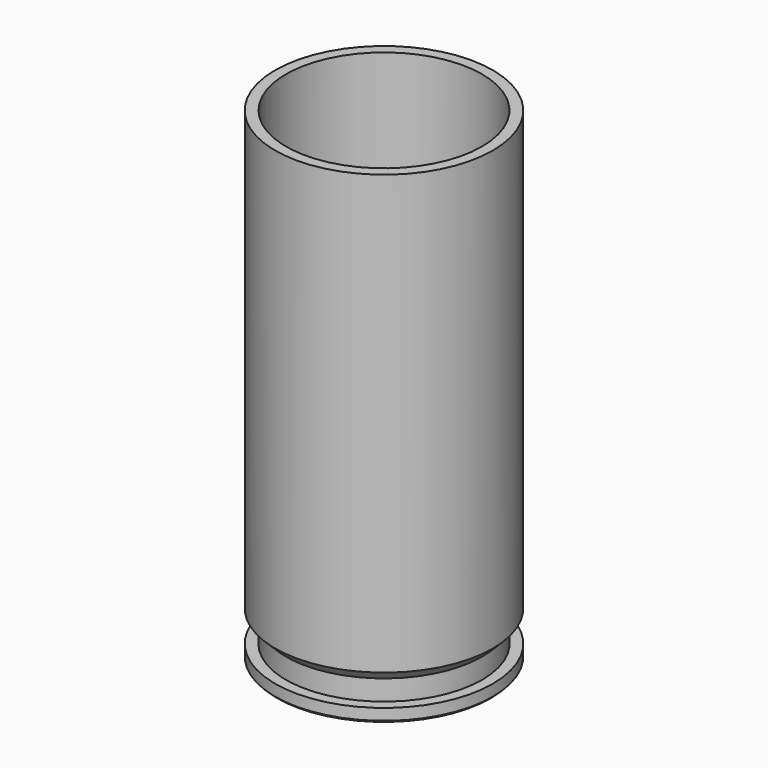
from build123d import *

# Parameters (mm, degrees)
F2_T        = -1.27
F3_SIZE     = 0.254
F4_R        = 6.9696549561
F4_R_2      = 6.3199888533
F5_DEPTH    = 0.254
F7_S5_R     = 11.5270866081
F7_T6_DEPTH = 20


# Not quite as in the source:
# - a fillet or chamfer that OpenCascade refuses, or shapes differently, is made with other operations: its cross-section is extruded or revolved along the edge and cut away or added


with BuildPart() as f1:
    # F0 (on Front) → F1 (revolve)
    with BuildSketch(Plane.XZ):
        Polygon((0, 56.7248165607), (0, 0), (12.7805937082, 0), (12.7805937082, 1.5856500249), (11.5270866081, 1.5856500249), (11.5270866081, 2.6958733797), (12.7805937082, 2.6958733797), (12.7805937082, 56.7248165607), align=None)
    revolve(axis=Axis((0, 0, 24.1605676711), (0, 0, -1)))

    # F2
    f2_openings = [f1.faces().sort_by_distance(p)[0] for p in [
        (0, 0, 56.724817),
    ]]
    offset(amount=F2_T, openings=f2_openings, kind=Kind.INTERSECTION)

    # F3
    f3_edges = [f1.edges().sort_by_distance(p)[0] for p in [
        (-12.780594, 0, 0),
    ]]
    chamfer(f3_edges, length=F3_SIZE)

    # F4 (on face) → F5 (cut)
    with BuildSketch(Plane(origin=(0, 0, 0), x_dir=(1, 0, 0), z_dir=(0, 0, -1))):
        Circle(F4_R)
        Circle(F4_R_2, mode=Mode.SUBTRACT)
    extrude(amount=-F5_DEPTH, mode=Mode.SUBTRACT)

    # F6: fillet of radius 0.762 on 2 edges, made by hand

    # F6_s1 → F6_t2 (revolve, cut)
    with BuildSketch(Plane.XZ):
        with BuildLine():
            ThreePointArc((6.3199888533, 0.254), (6.0631127843, 0.066392352), (5.752027587, 0))
            Line((5.752027587, 0), (6.3199888533, 0))
            Line((6.3199888533, 0), (6.3199888533, 0.254))
        make_face()
    revolve(axis=Axis((0, 0, 0), (0, 0, -1)), mode=Mode.SUBTRACT)

    # F6_s3 → F6_t4 (revolve, cut)
    with BuildSketch(Plane.XZ):
        with BuildLine():
            ThreePointArc((7.5376162224, 0), (7.226531025, 0.066392352), (6.9696549561, 0.254))
            Line((6.9696549561, 0.254), (6.9696549561, 0))
            Line((6.9696549561, 0), (7.5376162224, 0))
        make_face()
    revolve(axis=Axis((0, 0, 0), (0, 0, -1)), mode=Mode.SUBTRACT)

    # F7: chamfer of 2.54 on 1 edges, made by hand


with BuildPart() as f7_tool2:
    # F7_s3 → F7_t4 (revolve)
    with BuildSketch(Plane.XZ):
        Polygon((10.2405937082, 2.6958733797), (12.7805937082, 5.2358733797), (12.7805937082, 2.6958733797), align=None)
    revolve(axis=Axis((0, 0, 2.6958733797), (0, 0, -1)))

    # F7_s5 → F7_t6 (cut, symmetric)
    with BuildSketch(Plane.XY.offset(4)):
        Circle(F7_S5_R)
    extrude(amount=F7_T6_DEPTH, both=True, mode=Mode.SUBTRACT)


with BuildPart() as f1_1:
    add(f1.part)

    # F7_t1: cut F7_tool2
    add(f7_tool2.part, mode=Mode.SUBTRACT)


solid = f1_1.part
